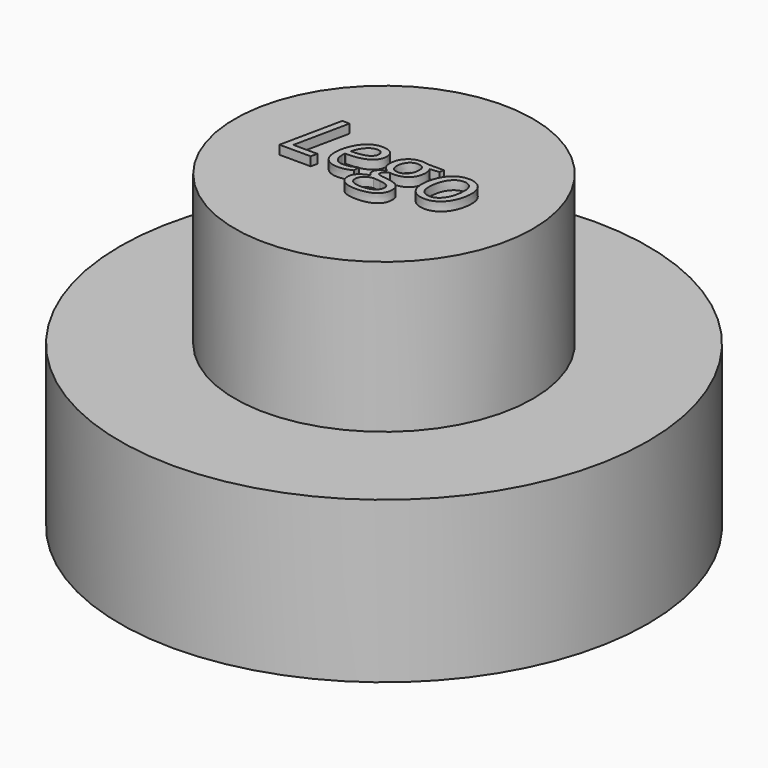
from build123d import *

# Parameters (mm, degrees)
F0_R         = 6.0507692662
F1_DEPTH     = 3.683
F2_R         = 3.4157704239
F3_DEPTH     = 3.429
F4_R         = 3.1658634543
F5_DEPTH     = 2.794
F6_TEXT_SIZE = 1.9962207362
F7_DEPTH     = 0.2032


# Not quite as in the source:
# - Text() gives the source's letters only with a copy of the font that has no kerning and outlines rounded to 1/6400 em; it was checked with that copy


with BuildPart() as f1:
    # F0 (on Top) → F1 (new body)
    with BuildSketch(Plane.XY):
        Circle(F0_R)
    extrude(amount=F1_DEPTH)

    # F2 (on face) → F3 (join)
    with BuildSketch(Plane.XY.offset(3.683)):
        Circle(F2_R)
    extrude(amount=F3_DEPTH)

    # F4 (on face) → F5 (cut)
    with BuildSketch(Plane(origin=(0, 0, 0), x_dir=(1, 0, 0), z_dir=(0, 0, -1))):
        Circle(F4_R)
    extrude(amount=-F5_DEPTH, mode=Mode.SUBTRACT)

    # F6 (on face) → F7 (join)
    with BuildSketch(Plane.XY.offset(7.112)):
        with Locations((-2.0052422187, -0.5940220435)):
            Text('Lego', F6_TEXT_SIZE, font='Open Sans', font_style=FontStyle.ITALIC, text_align=(TextAlign.LEFT, TextAlign.BOTTOM))
    extrude(amount=F7_DEPTH)


solid = f1.part
